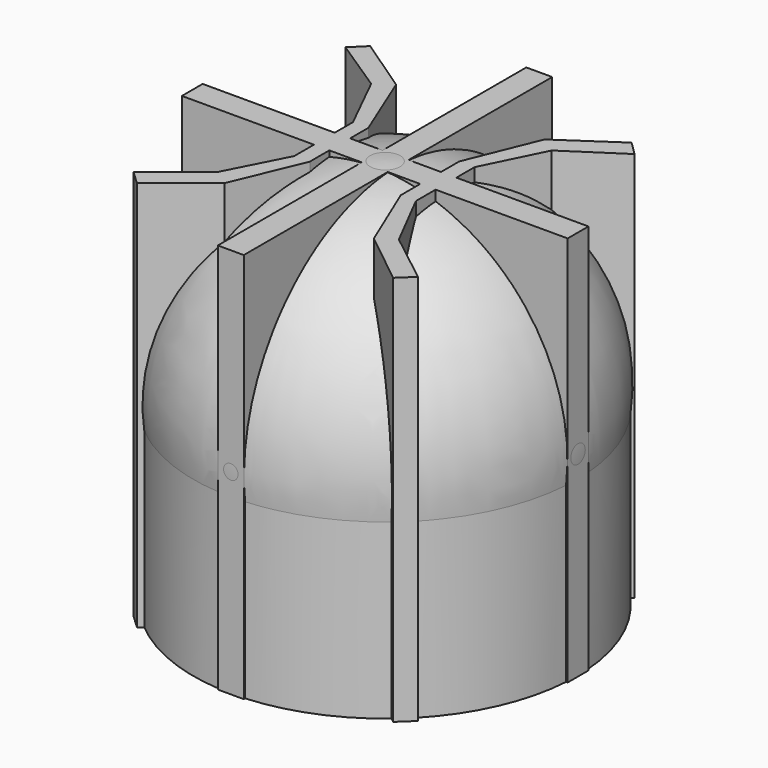
from build123d import *

# Parameters (mm, degrees)
F0_R     = 37.5
F3_DEPTH = 34.544
F4_W     = 2.54
F4_H     = 35.1937671816
F4_H_2   = 5.08
F4_W_2   = 25.8245437388
F4_H_3   = 35.1272260463
F5_DEPTH = 76.454


with BuildPart() as f2:
    # F1 (on Right) → F2 (revolve)
    with BuildSketch(Plane.YZ):
        with BuildLine():
            Line((0, 0), (0, 76.6080915928))
            ThreePointArc((0, 76.6080915928), (-37.7602969141, 38.3040457964), (0, 0))
        make_face()
    revolve(axis=Axis((0, 0, 0), (0, 0, 1)))

    # F0 (on Top) → F3 (join)
    with BuildSketch(Plane.XY):
        Circle(F0_R)
    extrude(amount=F3_DEPTH)

    # F4 (on Top) → F5 (join)
    with BuildSketch(Plane.XY):
        Polygon((14.625684157, -21.0453859377), (25.0486971238, -29.3630193568), (27.8219762537, -26.7505448847), (17.8159009493, -18.9295182894), align=None)
        Polygon((8.89, -7.2986403331), (14.625684157, -21.0453859377), (17.8159009493, -18.9295182894), (11.8944562612, -7.3510332484), align=None)
        Polygon((8.89, -2.54), (8.89, -7.2986403331), (11.8944562612, -7.3510332484), (11.8944562612, -2.54), align=None)
        Polygon((2.54, -2.54), (8.89, -2.54), (8.89, -0.3136403331), (8.89, 2.54), (2.54, 2.54), align=None)
        Polygon((8.89, -0.3136403331), (8.89, -2.54), (11.8944562612, -2.54), (11.8944562612, 2.54), (8.89, 2.54), align=None)
        with Locations((1.27, -20.1368835908)):
            Rectangle(F4_W, F4_H)
        with Locations((1.27, 0)):
            Rectangle(F4_W, F4_H_2)
        with Locations((24.8067281306, 0)):
            Rectangle(F4_W_2, F4_H_2)
        Polygon((8.89, 6.9984272738), (8.89, 2.54), (11.8944562612, 2.54), (11.8944562612, 6.9925217125), align=None)
        with Locations((-1.27, 0)):
            Rectangle(F4_W, F4_H_2)
        with Locations((-1.27, -20.1368835908)):
            Rectangle(F4_W, F4_H)
        with Locations((1.27, 20.1036130232)):
            Rectangle(F4_W, F4_H_3)
        Polygon((14.5159834457, 20.8089271088), (8.89, 6.9984272738), (11.8944562612, 6.9925217125), (17.6561749355, 18.6513132862), align=None)
        with Locations((-1.27, 20.1036130232)):
            Rectangle(F4_W, F4_H_3)
        Polygon((-8.89, -2.54), (-2.54, -2.54), (-2.54, 2.54), (-8.89, 2.54), (-8.89, -0.3136403331), align=None)
        Polygon((25.5505285726, 28.2963191009), (14.5159834457, 20.8089271088), (17.6561749355, 18.6513132862), (28.268991402, 25.626851018), align=None)
        Polygon((-11.8944562612, -2.54), (-8.89, -2.54), (-8.89, -0.3136403331), (-8.89, 2.54), (-11.8944562612, 2.54), align=None)
        Polygon((-8.89, -7.2986403331), (-8.89, -2.54), (-11.8944562612, -2.54), (-11.8944562612, -7.3510332484), align=None)
        Polygon((-11.8944562612, 2.54), (-8.89, 2.54), (-8.89, 6.9984272738), (-11.8944562612, 6.9925217125), align=None)
        Polygon((-14.625684157, -21.0453859377), (-8.89, -7.2986403331), (-11.8944562612, -7.3510332484), (-17.8159009493, -18.9295182894), align=None)
        with Locations((-24.8067281306, 0)):
            Rectangle(F4_W_2, F4_H_2)
        Polygon((-11.8944562612, 6.9925217125), (-8.89, 6.9984272738), (-14.5159834457, 20.8089271088), (-17.6561749355, 18.6513132862), align=None)
        Polygon((-25.0486971238, -29.3630193568), (-14.625684157, -21.0453859377), (-17.8159009493, -18.9295182894), (-27.8219762537, -26.7505448847), align=None)
        Polygon((-17.6561749355, 18.6513132862), (-14.5159834457, 20.8089271088), (-25.5505285726, 28.2963191009), (-28.268991402, 25.626851018), align=None)
    extrude(amount=F5_DEPTH)


solid = f2.part
